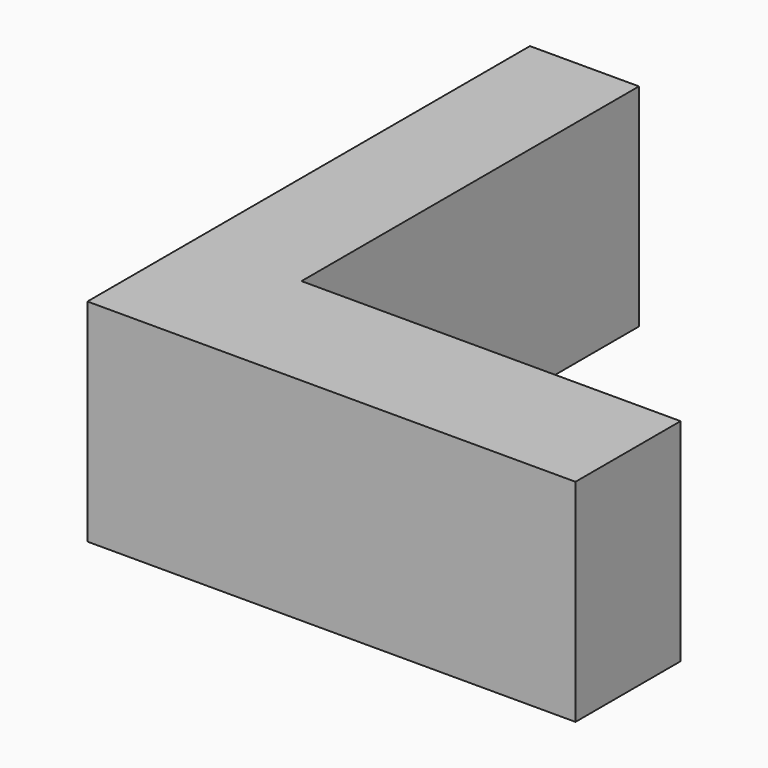
from build123d import *

# Parameters (mm, degrees)
F1_DEPTH = 25


# Not quite as in the source:
# - a feature names something its author has since deleted; it is built from what else it names


with BuildPart() as f1:
    # F0 (on Top) → F1 (new body)
    with BuildSketch(Plane.XY):
        Polygon((-10.947361527, 40.2089878917), (-23.8386318088, 40.2089878917), (-23.8386318088, -25.201132521), (33.87792781, -25.201132521), (33.87792781, -9.6702389419), (-10.947361527, -9.6702389419), align=None)
    extrude(amount=F1_DEPTH)


solid = f1.part
